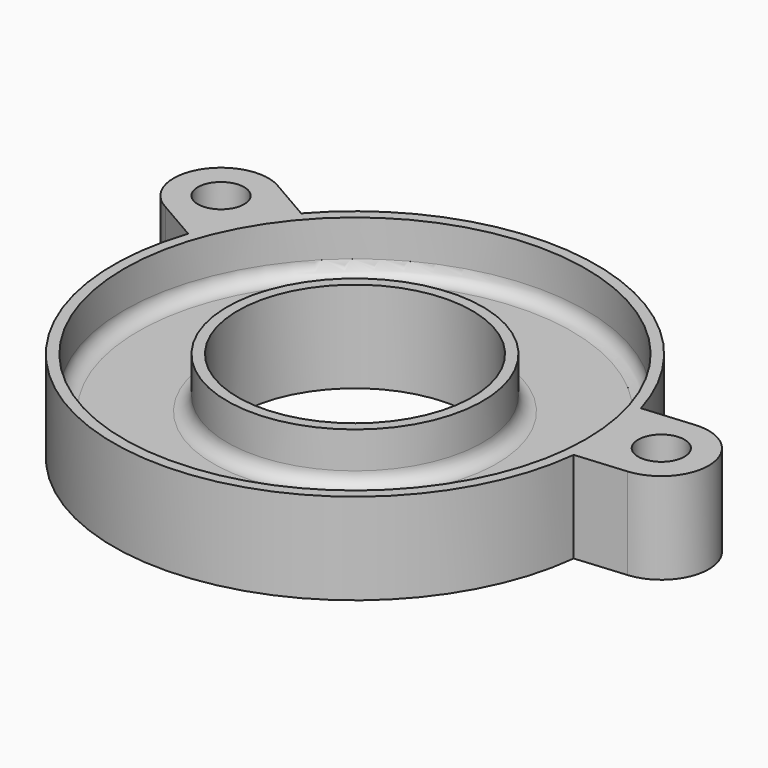
from build123d import *

# Parameters (mm, degrees)
F2_R     = 1.65
F3_DEPTH = 6.5
F4_SIZE  = 1.2
F5_R     = 1


# Not quite as in the source:
# - a feature names something its author has since deleted; it is built from what else it names


with BuildPart() as f1:
    # F0 (on Right) → F1 (revolve)
    with BuildSketch(Plane.YZ):
        Polygon((8.35, 0), (17.2, 0), (17.2, 6.5), (16.45, 6.5), (16.45, 2.9), (9.1, 2.9), (9.1, 6.5), (8.35, 6.5), align=None)
    revolve(axis=Axis((0, 0, -2.445915569), (0, 0, -1)))

    # F2 (on Top) → F3 (join, through all)
    with BuildSketch(Plane.XY):
        with BuildLine():
            Line((-12.9185614558, 11.3556492511), (-16.0443701425, 13.1603357378))
            ThreePointArc((-16.0443701425, 13.1603357378), (-20.6890755738, 11.8640180715), (-19.2967065825, 7.2471970193))
            Line((-19.2967065825, 7.2471970193), (-16.2926126828, 5.5127825977))
            ThreePointArc((-16.2926126828, 5.5127825977), (-14.8948966536, 8.6012820951), (-12.9185614558, 11.3556492511))
        make_face()
        with Locations((-17.7318701425, 10.2375)):
            Circle(F2_R, mode=Mode.SUBTRACT)
        with BuildLine():
            ThreePointArc((16.5081291827, 4.8292515868), (17.1346777754, 1.4976039307), (17.0955988557, -1.8922208557))
            Line((17.0955988557, -1.8922208557), (20.6912370752, -1.5776432733))
            ThreePointArc((20.6912370752, -1.5776432733), (23.752419757, 2.1483315823), (19.9637580849, 5.1315799411))
            Line((19.9637580849, 5.1315799411), (16.5081291827, 4.8292515868))
        make_face()
        with Locations((20.3970864434, 1.7845138328)):
            Circle(F2_R, mode=Mode.SUBTRACT)
    extrude(amount=F3_DEPTH)

    # F4
    f4_edges = [f1.edges().sort_by_distance(p)[0] for p in [
        (-19.38187, 10.2375, 0),
    ]]
    chamfer(f4_edges, length=F4_SIZE)

    # F5
    f5_edges = [f1.edges().sort_by_distance(p)[0] for p in [
        (0, -16.45, 2.9),
        (0, -9.1, 2.9),
    ]]
    fillet(f5_edges, radius=F5_R)


solid = f1.part
